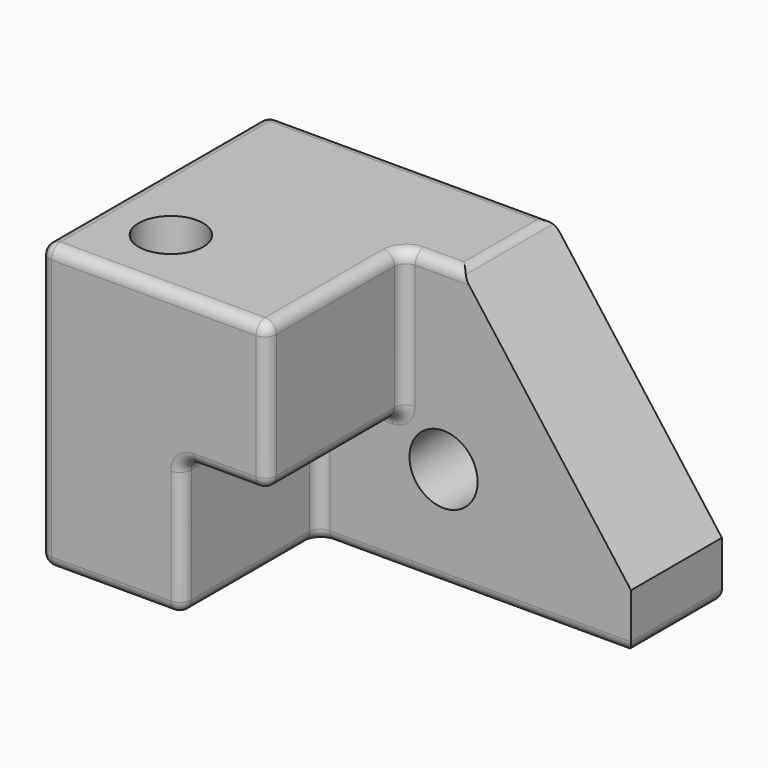
from build123d import *

# Parameters (mm, degrees)
F0_W     = 203.2
F0_H     = 127
F1_DEPTH = 127
F3_DEPTH = 76.2
F4_SIZE2 = 101.6
F4_SIZE  = 76.2
F5_R     = 5.08
F6_R     = 15.24
F7_DEPTH = 50.8
F8_R     = 14.4150748184
F9_DEPTH = 127


with BuildPart() as f1:
    # F0 (on Front) → F1 (new body)
    with BuildSketch(Plane.XZ):
        with Locations((-6.4546563804, 2.2225044668)):
            Rectangle(F0_W, F0_H)
    extrude(amount=F1_DEPTH)

    # F2 (on face) → F3 (cut)
    with BuildSketch(Plane.XZ.offset(127)):
        Polygon((95.1453436196, 65.7225044668), (-6.4546563804, 65.7225044668), (-6.4546563804, 0), (-44.5546563804, 0), (-44.5546563804, -61.2774955332), (95.1453436196, -61.2774955332), align=None)
    extrude(amount=-F3_DEPTH, mode=Mode.SUBTRACT)

    # F4
    f4_edges = [f1.edges().sort_by_distance(p)[0] for p in [
        (95.145344, -25.4, 65.722504),
    ]]
    f4_side = f1.faces().sort_by_distance((-28.226085, -52.614286, 65.722504))[0]
    chamfer(f4_edges, length=F4_SIZE, length2=F4_SIZE2, reference=f4_side)

    # F5
    f5_edges = [f1.edges().sort_by_distance(p)[0] for p in [
        (-6.454656, -88.9, 65.722504),
        (-57.254656, -127, 65.722504),
        (-6.454656, -127, 32.861252),
        (-6.454656, -88.9, 0),
        (-6.454656, -50.8, 32.861252),
        (18.945344, -25.4, 65.722504),
        (-44.554656, 0, 65.722504),
        (-108.054656, -63.5, 65.722504),
        (6.245344, -50.8, 65.722504),
        (-25.504656, -127, 0),
        (-44.554656, -127, -30.638748),
        (-76.304656, -127, -61.277496),
        (-108.054656, -127, 2.222504),
        (-44.554656, -88.9, 0),
        (-44.554656, -88.9, -61.277496),
        (-44.554656, -50.8, -30.638748),
        (-6.454656, 0, -61.277496),
        (95.145344, -25.4, -61.277496),
        (25.295344, -50.8, -61.277496),
        (-108.054656, -63.5, -61.277496),
        (-108.054656, 0, 2.222504),
        (-25.504656, -50.8, 0),
    ]]
    fillet(f5_edges, radius=F5_R)

    # F6 (on face) → F7 (cut, through all)
    with BuildSketch(Plane.XZ.offset(50.8)):
        with Locations((11.3253436196, -15.5574955332)):
            Circle(F6_R)
    extrude(amount=-F7_DEPTH, mode=Mode.SUBTRACT)

    # F8 (on face) → F9 (cut, through all)
    with BuildSketch(Plane.XY.offset(65.7225044668)):
        with Locations((-76.158054173, -93.8184931874)):
            Circle(F8_R)
    extrude(amount=-F9_DEPTH, mode=Mode.SUBTRACT)


solid = f1.part
